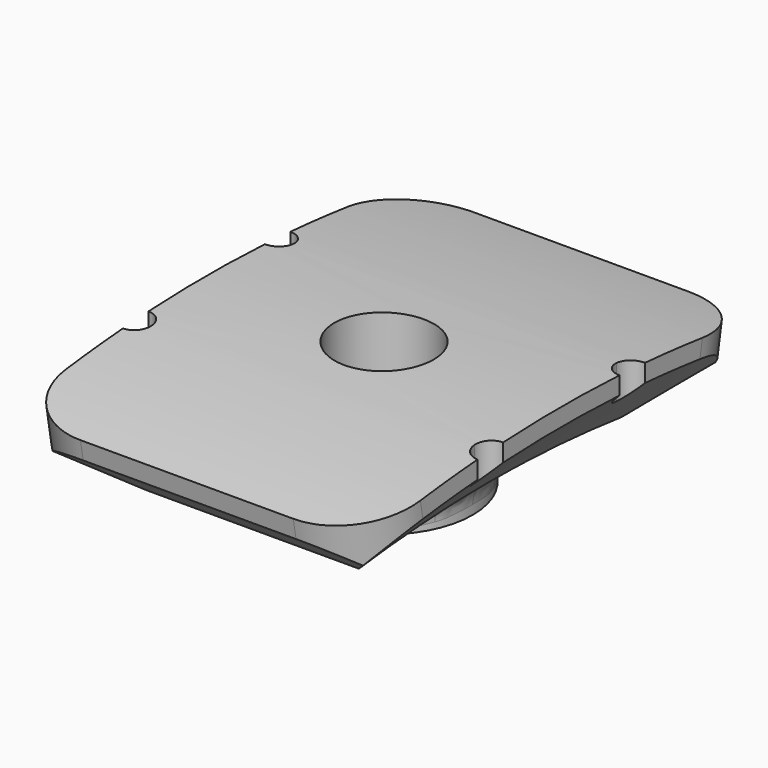
from build123d import *

# Parameters (mm, degrees)
F1_DEPTH    = 12.7
F2_R        = 3.556
F3_DEPTH    = 25.4
F4_DEPTH    = 25.4
F5_T1_DEPTH = 50.9025417293
F5_T4_ANGLE = 21.9844621663
F5_T6_ANGLE = 21.9844621663
F7_R        = 6.35
F7_R_2      = 3.556
F8_DEPTH    = 2.54
F10_R       = 2.032
F11_R       = 5.08


# Not quite as in the source:
# - a fillet or chamfer that OpenCascade refuses, or shapes differently, is made with other operations: its cross-section is extruded or revolved along the edge and cut away or added


with BuildPart() as f1:
    # F0 (on Right) → F1 (new body, symmetric)
    with BuildSketch(Plane.YZ):
        with BuildLine():
            Line((16.5399889228, -7.7970615256), (17.642654851, -1.543532294))
            ThreePointArc((17.642654851, -1.543532294), (0, 0), (-17.642654851, -1.543532294))
            Line((-17.642654851, -1.543532294), (-16.5399889228, -7.7970615256))
            ThreePointArc((-16.5399889228, -7.7970615256), (0, -6.35), (16.5399889228, -7.7970615256))
        make_face()
    extrude(amount=F1_DEPTH, both=True)

    # F2 (on Top) → F3 (cut)
    with BuildSketch(Plane.XY):
        Circle(F2_R)
    extrude(amount=-F3_DEPTH, mode=Mode.SUBTRACT)

    # F2 (on Top) → F4 (cut)
    with BuildSketch(Plane.XY):
        with BuildLine():
            Line((-12.7, 6.35), (-11.557, 6.35))
            ThreePointArc((-11.557, 6.35), (-13.5082230509, 7.1582230509), (-12.7, 5.207))
            Line((-12.7, 5.207), (-12.7, 6.35))
        make_face()
        with BuildLine():
            ThreePointArc((-12.7, 5.207), (-11.8917769491, 5.5417769491), (-11.557, 6.35))
            Line((-11.557, 6.35), (-12.7, 6.35))
            Line((-12.7, 6.35), (-12.7, 5.207))
        make_face()
        with BuildLine():
            ThreePointArc((13.843, 6.35), (12.7, 7.493), (11.557, 6.35))
            Line((11.557, 6.35), (12.7, 6.35))
            Line((12.7, 6.35), (12.7, 5.207))
            ThreePointArc((12.7, 5.207), (13.5082230509, 5.5417769491), (13.843, 6.35))
        make_face()
        with BuildLine():
            Line((12.7, 6.35), (11.557, 6.35))
            ThreePointArc((11.557, 6.35), (11.8917769491, 5.5417769491), (12.7, 5.207))
            Line((12.7, 5.207), (12.7, 6.35))
        make_face()
        with BuildLine():
            Line((-12.7, -6.35), (-12.7, -5.207))
            ThreePointArc((-12.7, -5.207), (-13.5082230509, -7.1582230509), (-11.557, -6.35))
            Line((-11.557, -6.35), (-12.7, -6.35))
        make_face()
        with BuildLine():
            ThreePointArc((-11.557, -6.35), (-11.8917769491, -5.5417769491), (-12.7, -5.207))
            Line((-12.7, -5.207), (-12.7, -6.35))
            Line((-12.7, -6.35), (-11.557, -6.35))
        make_face()
        with BuildLine():
            ThreePointArc((13.843, -6.35), (13.5082230509, -5.5417769491), (12.7, -5.207))
            Line((12.7, -5.207), (12.7, -6.35))
            Line((12.7, -6.35), (11.557, -6.35))
            ThreePointArc((11.557, -6.35), (12.7, -7.493), (13.843, -6.35))
        make_face()
        with BuildLine():
            Line((12.7, -6.35), (12.7, -5.207))
            ThreePointArc((12.7, -5.207), (11.8917769491, -5.5417769491), (11.557, -6.35))
            Line((11.557, -6.35), (12.7, -6.35))
        make_face()
    extrude(amount=-F4_DEPTH, mode=Mode.SUBTRACT)

    # F5: chamfer of 5.08 on 4 edges, made by hand

    # F5_s2 → F5_t1 (cut)
    with BuildSketch(Plane.YZ.offset(-25.4512708646)):
        with BuildLine():
            Line((-11.7692577282, -7.0799118043), (-17.3997748591, -2.9209731764))
            Line((-17.3997748591, -2.9209731764), (-16.5399889228, -7.7970615256))
            ThreePointArc((-16.5399889228, -7.7970615256), (-14.0880401184, -7.3976134823), (-11.7692577282, -7.0799118043))
        make_face()
        with BuildLine():
            Line((11.7692577282, -7.0799118043), (17.3997748591, -2.9209731764))
            Line((17.3997748591, -2.9209731764), (16.5399889228, -7.7970615256))
            ThreePointArc((16.5399889228, -7.7970615256), (14.0880401184, -7.3976134823), (11.7692577282, -7.0799118043))
        make_face()
    extrude(amount=F5_T1_DEPTH, mode=Mode.SUBTRACT)

    # F5_s3 → F5_t4 (revolve, cut)
    with BuildSketch(Plane(origin=(0, -19.0172411137, -3.6939012396), x_dir=(1, 0, 0), z_dir=(0, -0.9816530468, -0.1906758917))):
        Polygon((-7.62, -4.4859495571), (-12.7, 0.5940504429), (-12.7, -4.4859495571), align=None)
    revolve(axis=Axis((-12.7, 0, -101.6), (-1, 0, 0)), revolution_arc=F5_T4_ANGLE, mode=Mode.SUBTRACT)

    # F5_s5 → F5_t6 (revolve, cut)
    with BuildSketch(Plane(origin=(0, -19.0172411137, -3.6939012396), x_dir=(1, 0, 0), z_dir=(0, -0.9816530468, -0.1906758917))):
        Polygon((7.62, -4.4859495571), (12.7, 0.5940504429), (12.7, -4.4859495571), align=None)
    revolve(axis=Axis((12.7, 0, -101.6), (-1, 0, 0)), revolution_arc=F5_T6_ANGLE, mode=Mode.SUBTRACT)

    # F7 (on offset) → F8 (join)
    with BuildSketch(Plane.XY.offset(-6.35)):
        Circle(F7_R)
        Circle(F7_R_2, mode=Mode.SUBTRACT)
    extrude(amount=-F8_DEPTH)

    # F9: union 

    # F10
    f10_edges = [f1.edges().sort_by_distance(p)[0] for p in [
        (-6.35, 0, -6.35),
    ]]
    fillet(f10_edges, radius=F10_R)

    # F11
    f11_edges = [f1.edges().sort_by_distance(p)[0] for p in [
        (12.7, 17.532388, -2.168885),
        (-12.7, 17.532388, -2.168885),
        (12.7, -17.532388, -2.168885),
        (-12.7, -17.532388, -2.168885),
    ]]
    fillet(f11_edges, radius=F11_R)


solid = f1.part
